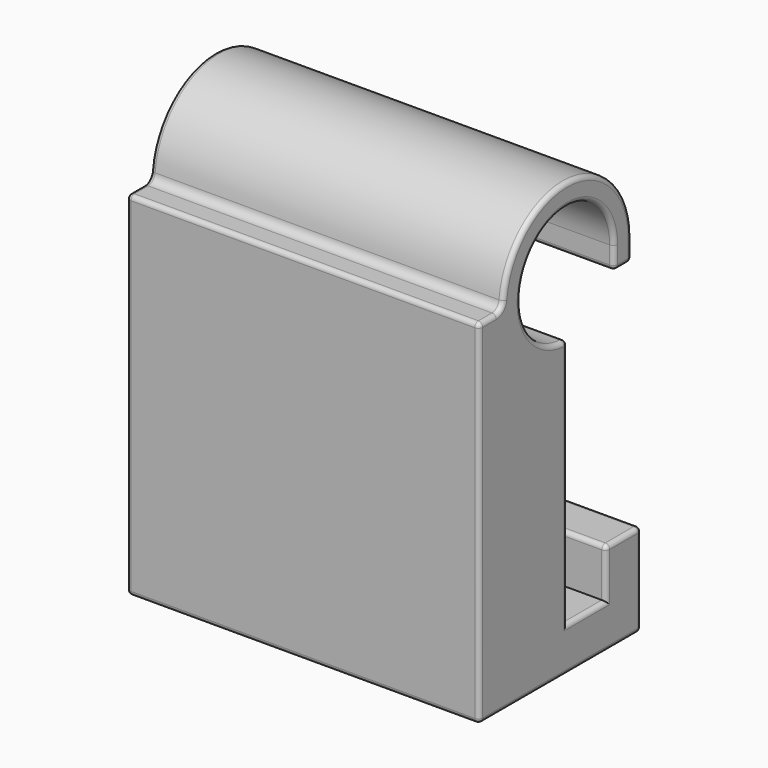
from build123d import *

# Parameters (mm, degrees)
F1_DEPTH = 40
F2_W     = 5.5
F2_H     = 5.5
F3_DEPTH = 11
F4_R     = 2
F5_R     = 1


# Not quite as in the source:
# - a feature names something its author has since deleted; it is built from what else it names


with BuildPart() as f1:
    # F0 (on Right) → F1 (new body, symmetric)
    with BuildSketch(Plane.YZ):
        with BuildLine():
            ThreePointArc((0, -18.25), (-12.9046987567, -12.9046987567), (-18.25, 0))
            Line((-18.25, 0), (-25, 0))
            Line((-25, 0), (-25, -80))
            Line((-25, -80), (21, -80))
            Line((21, -80), (21, -59))
            Line((21, -59), (11, -59))
            Line((11, -59), (11, -70))
            Line((11, -70), (0, -70))
            Line((0, -70), (0, -18.25))
        make_face()
        with BuildLine():
            Line((-13.25, 0), (-18.25, 0))
            ThreePointArc((-18.25, 0), (-12.9046987567, -12.9046987567), (0, -18.25))
            Line((0, -18.25), (0, -13.25))
            ThreePointArc((0, -13.25), (-9.3691648507, -9.3691648507), (-13.25, 0))
        make_face()
        with BuildLine():
            ThreePointArc((17.5517093185, -5), (18.0745842976, -2.5242627575), (18.25, 0))
            Line((18.25, 0), (13.25, 0))
            Line((13.25, 0), (13.25, -5))
            Line((13.25, -5), (17.5517093185, -5))
        make_face()
        with BuildLine():
            Line((18.25, -5), (18.25, 0))
            ThreePointArc((18.25, 0), (18.0745842976, -2.5242627575), (17.5517093185, -5))
            Line((17.5517093185, -5), (18.25, -5))
        make_face()
        with BuildLine():
            Line((13.25, 0), (18.25, 0))
            ThreePointArc((18.25, 0), (0, 18.25), (-18.25, 0))
            Line((-18.25, 0), (-13.25, 0))
            ThreePointArc((-13.25, 0), (0, 13.25), (13.25, 0))
        make_face()
    extrude(amount=F1_DEPTH, both=True)

    # F2 (on face) → F3 (cut)
    with BuildSketch(Plane(origin=(0, 0, 0), x_dir=(-1, 0, 0), z_dir=(0, 1, 0))):
        with Locations((-17.25, -29.25)):
            Rectangle(F2_W, F2_H)
        with Locations((-22.75, -29.25)):
            Rectangle(F2_W, F2_H)
        Polygon((-14.5, -32), (-20, -32), (-25.5, -32), (-25.5, -37.5), (-20, -37.5), (-14.5, -37.5), align=None)
        Polygon((25.5, -26.5), (20, -26.5), (14.5, -26.5), (14.5, -32), (14.5, -37.5), (20, -37.5), (25.5, -37.5), (25.5, -32), align=None)
    extrude(amount=-F3_DEPTH, mode=Mode.SUBTRACT)

    # F4
    f4_edges = [f1.edges().sort_by_distance(p)[0] for p in [
        (0, -18.25, 0),
    ]]
    fillet(f4_edges, radius=F4_R)

    # F5
    f5_edges = [f1.edges().sort_by_distance(p)[0] for p in [
        (-40, 0.902338, 18.227679),
        (-40, -18.808432, 0.517593),
        (-40, 18.25, -2.5),
        (-40, -22.575496, 0),
        (-40, 15.75, -5),
        (-40, -25, -40),
        (-40, 13.25, -2.5),
        (-40, -2, -80),
        (-40, -9.369165, 9.369165),
        (-40, 21, -69.5),
        (-40, 0, -41.625),
        (-40, 16, -59),
        (-40, 5.5, -70),
        (-40, 11, -64.5),
        (0, -25, -80),
        (40, -25, -40),
        (0, -25, 0),
        (40, 0.902338, 18.227679),
        (40, -18.808432, 0.517593),
        (40, 18.25, -2.5),
        (40, -22.575496, 0),
        (40, 15.75, -5),
        (40, 13.25, -2.5),
        (40, -2, -80),
        (40, -9.369165, 9.369165),
        (40, 21, -69.5),
        (40, 0, -41.625),
        (40, 16, -59),
        (40, 5.5, -70),
        (40, 11, -64.5),
        (0, 21, -80),
        (0, 21, -59),
        (0, 11, -59),
        (0, 18.25, -5),
        (0, 13.25, -5),
        (0, 0, -13.25),
        (25.5, 0, -32),
        (20, 0, -26.5),
        (14.5, 0, -32),
        (20, 0, -37.5),
        (-14.5, 0, -32),
        (-20, 0, -26.5),
        (-25.5, 0, -32),
        (-20, 0, -37.5),
    ]]
    fillet(f5_edges, radius=F5_R)


solid = f1.part
